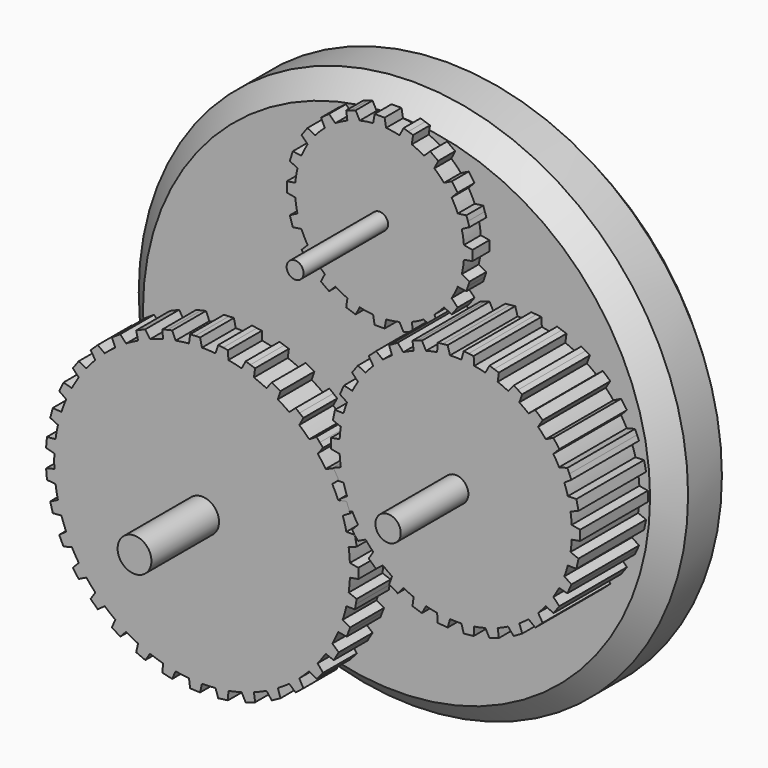
from build123d import *

# Parameters (mm, degrees)
F0_R      = 65
F1_DEPTH  = 20
F2_R      = 2
F3_DEPTH  = 5
F4_R      = 2
F5_DEPTH  = 30
F6_R      = 3
F7_DEPTH  = 20
F8_R      = 3
F9_DEPTH  = 40
F11_R     = 4
F12_DEPTH = 10
F13_R     = 4
F14_DEPTH = 40
F15_SIZE  = 5
F16_R     = 4
F17_DEPTH = 20
F18_DEPTH = 30
F19_W     = 40
F19_H     = 15
F20_DEPTH = 5
F21_W     = 8
F21_H     = 5
F22_DEPTH = 50
F24_DEPTH = 5
F26_DEPTH = 5
F27_W     = 10
F27_H     = 10
F28_DEPTH = 4
F29_DEPTH = 10
F30_R     = 2
F31_DEPTH = 4
F32_R     = 3
F33_DEPTH = 4


with BuildPart() as f1:
    # F0 (on Front) → F1 (new body)
    with BuildSketch(Plane.XZ):
        Circle(F0_R)
    extrude(amount=F1_DEPTH)

    # F15
    f15_edges = [f1.edges().sort_by_distance(p)[0] for p in [
        (-65, 0, 0),
        (65, -10, 0),
        (-65, -20, 0),
    ]]
    chamfer(f15_edges, length=F15_SIZE)

    # F16 (on face) → F17 (cut)
    with BuildSketch(Plane.XZ.offset(20)):
        with Locations((-30, -25)):
            Circle(F16_R)
    extrude(amount=-F17_DEPTH, mode=Mode.SUBTRACT)

    # F27 (on face) → F28 (cut)
    with BuildSketch(Plane(origin=(0, 0, 0), x_dir=(-1, 0, 0), z_dir=(0, 1, 0))):
        with Locations((-45, 0)):
            Rectangle(F27_W, F27_H)
        Polygon((-15.6698729811, -37.1410161514), (-24.3301270189, -32.1410161514), (-29.3301270189, -40.8012701892), (-20.6698729811, -45.8012701892), align=None)
        Polygon((24.3301270189, -32.1410161514), (15.6698729811, -37.1410161514), (20.6698729811, -45.8012701892), (29.3301270189, -40.8012701892), align=None)
        with Locations((45, 0)):
            Rectangle(F27_W, F27_H)
        Polygon((15.6698729811, 37.1410161514), (24.3301270189, 32.1410161514), (29.3301270189, 40.8012701892), (20.6698729811, 45.8012701892), align=None)
        Polygon((-24.3301270189, 32.1410161514), (-15.6698729811, 37.1410161514), (-20.6698729811, 45.8012701892), (-29.3301270189, 40.8012701892), align=None)
    extrude(amount=-F28_DEPTH, mode=Mode.SUBTRACT)


with BuildPart() as f3:
    # F2 (on face) → F3 (new body)
    with BuildSketch(Plane.XZ.offset(20)):
        with BuildLine():
            ThreePointArc((19.9409690564, 38.4645023307), (19.9852368153, 39.2316840258), (20, 40))
            ThreePointArc((20, 40), (19.9852368153, 40.7683159742), (19.9409690564, 41.5354976693))
            ThreePointArc((19.9409690564, 41.5354976693), (19.7537668119, 43.1286893008), (19.4394834369, 44.7017532586))
            ThreePointArc((19.4394834369, 44.7017532586), (19.0211303259, 46.1803398875), (18.4904936877, 47.6224433869))
            ThreePointArc((18.4904936877, 47.6224433869), (17.8201304838, 49.0798099948), (17.0351257359, 50.4787638185))
            ThreePointArc((17.0351257359, 50.4787638185), (16.1803398875, 51.7557050458), (15.230039966, 52.963251237))
            ThreePointArc((15.230039966, 52.963251237), (14.1421356237, 54.1421356237), (12.963251237, 55.230039966))
            ThreePointArc((12.963251237, 55.230039966), (11.7557050458, 56.1803398875), (10.4787638185, 57.0351257359))
            ThreePointArc((10.4787638185, 57.0351257359), (9.0798099948, 57.8201304838), (7.6224433869, 58.4904936877))
            ThreePointArc((7.6224433869, 58.4904936877), (6.1803398875, 59.0211303259), (4.7017532586, 59.4394834369))
            ThreePointArc((4.7017532586, 59.4394834369), (3.1286893008, 59.7537668119), (1.5354976693, 59.9409690564))
            ThreePointArc((1.5354976693, 59.9409690564), (0, 60), (-1.5354976693, 59.9409690564))
            ThreePointArc((-1.5354976693, 59.9409690564), (-3.1286893008, 59.7537668119), (-4.7017532586, 59.4394834369))
            ThreePointArc((-4.7017532586, 59.4394834369), (-6.1803398875, 59.0211303259), (-7.6224433869, 58.4904936877))
            ThreePointArc((-7.6224433869, 58.4904936877), (-9.0798099948, 57.8201304838), (-10.4787638185, 57.0351257359))
            ThreePointArc((-10.4787638185, 57.0351257359), (-11.7557050458, 56.1803398875), (-12.963251237, 55.230039966))
            ThreePointArc((-12.963251237, 55.230039966), (-14.1421356237, 54.1421356237), (-15.230039966, 52.963251237))
            ThreePointArc((-15.230039966, 52.963251237), (-16.1803398875, 51.7557050458), (-17.0351257359, 50.4787638185))
            ThreePointArc((-17.0351257359, 50.4787638185), (-17.8201304838, 49.0798099948), (-18.4904936877, 47.6224433869))
            ThreePointArc((-18.4904936877, 47.6224433869), (-19.0211303259, 46.1803398875), (-19.4394834369, 44.7017532586))
            ThreePointArc((-19.4394834369, 44.7017532586), (-19.7537668119, 43.1286893008), (-19.9409690564, 41.5354976693))
            ThreePointArc((-19.9409690564, 41.5354976693), (-20, 40), (-19.9409690564, 38.4645023307))
            ThreePointArc((-19.9409690564, 38.4645023307), (-19.7537668119, 36.8713106992), (-19.4394834369, 35.2982467414))
            ThreePointArc((-19.4394834369, 35.2982467414), (-19.0211303259, 33.8196601125), (-18.4904936877, 32.3775566131))
            ThreePointArc((-18.4904936877, 32.3775566131), (-17.8201304838, 30.9201900052), (-17.0351257359, 29.5212361815))
            ThreePointArc((-17.0351257359, 29.5212361815), (-16.1803398875, 28.2442949542), (-15.230039966, 27.036748763))
            ThreePointArc((-15.230039966, 27.036748763), (-14.1421356237, 25.8578643763), (-12.963251237, 24.769960034))
            ThreePointArc((-12.963251237, 24.769960034), (-11.7557050458, 23.8196601125), (-10.4787638185, 22.9648742641))
            ThreePointArc((-10.4787638185, 22.9648742641), (-9.0798099948, 22.1798695162), (-7.6224433869, 21.5095063123))
            ThreePointArc((-7.6224433869, 21.5095063123), (-6.1803398875, 20.9788696741), (-4.7017532586, 20.5605165631))
            ThreePointArc((-4.7017532586, 20.5605165631), (-3.1286893008, 20.2462331881), (-1.5354976693, 20.0590309436))
            ThreePointArc((-1.5354976693, 20.0590309436), (0, 20), (1.5354976693, 20.0590309436))
            ThreePointArc((1.5354976693, 20.0590309436), (3.1286893008, 20.2462331881), (4.7017532586, 20.5605165631))
            ThreePointArc((4.7017532586, 20.5605165631), (6.1803398875, 20.9788696741), (7.6224433869, 21.5095063123))
            ThreePointArc((7.6224433869, 21.5095063123), (9.0798099948, 22.1798695162), (10.4787638185, 22.9648742641))
            ThreePointArc((10.4787638185, 22.9648742641), (11.7557050458, 23.8196601125), (12.963251237, 24.769960034))
            ThreePointArc((12.963251237, 24.769960034), (14.1421356237, 25.8578643763), (15.230039966, 27.036748763))
            ThreePointArc((15.230039966, 27.036748763), (16.1803398875, 28.2442949542), (17.0351257359, 29.5212361815))
            ThreePointArc((17.0351257359, 29.5212361815), (17.8201304838, 30.9201900052), (18.4904936877, 32.3775566131))
            ThreePointArc((18.4904936877, 32.3775566131), (19.0211303259, 33.8196601125), (19.4394834369, 35.2982467414))
            ThreePointArc((19.4394834369, 35.2982467414), (19.7537668119, 36.8713106992), (19.9409690564, 38.4645023307))
        make_face()
        with Locations((0, 40)):
            Circle(F2_R, mode=Mode.SUBTRACT)
        with BuildLine():
            ThreePointArc((19.9409690564, 41.5354976693), (19.9852368153, 40.7683159742), (20, 40))
            ThreePointArc((20, 40), (19.9852368153, 39.2316840258), (19.9409690564, 38.4645023307))
            Line((19.9409690564, 38.4645023307), (21.9684390888, 38.822))
            Line((21.9684390888, 38.822), (21.9684390888, 40))
            Line((21.9684390888, 40), (21.9684390888, 41.178))
            Line((21.9684390888, 41.178), (19.9409690564, 41.5354976693))
        make_face()
        with BuildLine():
            ThreePointArc((18.4904936877, 47.6224433869), (19.0211303259, 46.1803398875), (19.4394834369, 44.7017532586))
            Line((19.4394834369, 44.7017532586), (21.2572491676, 45.6682764421))
            Line((21.2572491676, 45.6682764421), (20.8932271483, 46.7886210183))
            Line((20.8932271483, 46.7886210183), (20.5292051289, 47.9089655945))
            Line((20.5292051289, 47.9089655945), (18.4904936877, 47.6224433869))
        make_face()
        with BuildLine():
            Line((21.2572491676, 34.3317235579), (19.4394834369, 35.2982467414))
            ThreePointArc((19.4394834369, 35.2982467414), (19.0211303259, 33.8196601125), (18.4904936877, 32.3775566131))
            Line((18.4904936877, 32.3775566131), (20.5292051289, 32.0910344055))
            Line((20.5292051289, 32.0910344055), (20.8932271483, 33.2113789817))
            Line((20.8932271483, 33.2113789817), (21.2572491676, 34.3317235579))
        make_face()
        with BuildLine():
            ThreePointArc((15.230039966, 52.963251237), (16.1803398875, 51.7557050458), (17.0351257359, 50.4787638185))
            Line((17.0351257359, 50.4787638185), (18.46525159, 51.9597024929))
            Line((18.46525159, 51.9597024929), (17.7728405628, 52.9127245123))
            Line((17.7728405628, 52.9127245123), (17.0804295356, 53.8657465317))
            Line((17.0804295356, 53.8657465317), (15.230039966, 52.963251237))
        make_face()
        with BuildLine():
            Line((18.46525159, 28.0402975071), (17.0351257359, 29.5212361815))
            ThreePointArc((17.0351257359, 29.5212361815), (16.1803398875, 28.2442949542), (15.230039966, 27.036748763))
            Line((15.230039966, 27.036748763), (17.0804295356, 26.1342534683))
            Line((17.0804295356, 26.1342534683), (17.7728405628, 27.0872754877))
            Line((17.7728405628, 27.0872754877), (18.46525159, 28.0402975071))
        make_face()
        with BuildLine():
            ThreePointArc((10.4787638185, 57.0351257359), (11.7557050458, 56.1803398875), (12.963251237, 55.230039966))
            Line((12.963251237, 55.230039966), (13.8657465317, 57.0804295356))
            Line((13.8657465317, 57.0804295356), (12.9127245123, 57.7728405628))
            Line((12.9127245123, 57.7728405628), (11.9597024929, 58.46525159))
            Line((11.9597024929, 58.46525159), (10.4787638185, 57.0351257359))
        make_face()
        with BuildLine():
            Line((13.8657465317, 22.9195704644), (12.963251237, 24.769960034))
            ThreePointArc((12.963251237, 24.769960034), (11.7557050458, 23.8196601125), (10.4787638185, 22.9648742641))
            Line((10.4787638185, 22.9648742641), (11.9597024929, 21.53474841))
            Line((11.9597024929, 21.53474841), (12.9127245123, 22.2271594372))
            Line((12.9127245123, 22.2271594372), (13.8657465317, 22.9195704644))
        make_face()
        with BuildLine():
            ThreePointArc((4.7017532586, 59.4394834369), (6.1803398875, 59.0211303259), (7.6224433869, 58.4904936877))
            Line((7.6224433869, 58.4904936877), (7.9089655945, 60.5292051289))
            Line((7.9089655945, 60.5292051289), (6.7886210183, 60.8932271483))
            Line((6.7886210183, 60.8932271483), (5.6682764421, 61.2572491676))
            Line((5.6682764421, 61.2572491676), (4.7017532586, 59.4394834369))
        make_face()
        with BuildLine():
            Line((7.9089655945, 19.4707948711), (7.6224433869, 21.5095063123))
            ThreePointArc((7.6224433869, 21.5095063123), (6.1803398875, 20.9788696741), (4.7017532586, 20.5605165631))
            Line((4.7017532586, 20.5605165631), (5.6682764421, 18.7427508324))
            Line((5.6682764421, 18.7427508324), (6.7886210183, 19.1067728517))
            Line((6.7886210183, 19.1067728517), (7.9089655945, 19.4707948711))
        make_face()
        with BuildLine():
            ThreePointArc((-1.5354976693, 59.9409690564), (0, 60), (1.5354976693, 59.9409690564))
            Line((1.5354976693, 59.9409690564), (1.178, 61.9684390888))
            Line((1.178, 61.9684390888), (0, 61.9684390888))
            Line((0, 61.9684390888), (-1.178, 61.9684390888))
            Line((-1.178, 61.9684390888), (-1.5354976693, 59.9409690564))
        make_face()
        with BuildLine():
            Line((1.178, 18.0315609112), (1.5354976693, 20.0590309436))
            ThreePointArc((1.5354976693, 20.0590309436), (0, 20), (-1.5354976693, 20.0590309436))
            Line((-1.5354976693, 20.0590309436), (-1.178, 18.0315609112))
            Line((-1.178, 18.0315609112), (0, 18.0315609112))
            Line((0, 18.0315609112), (1.178, 18.0315609112))
        make_face()
        with BuildLine():
            ThreePointArc((-7.6224433869, 58.4904936877), (-6.1803398875, 59.0211303259), (-4.7017532586, 59.4394834369))
            Line((-4.7017532586, 59.4394834369), (-5.6682764421, 61.2572491676))
            Line((-5.6682764421, 61.2572491676), (-6.7886210183, 60.8932271483))
            Line((-6.7886210183, 60.8932271483), (-7.9089655945, 60.5292051289))
            Line((-7.9089655945, 60.5292051289), (-7.6224433869, 58.4904936877))
        make_face()
        with BuildLine():
            Line((-5.6682764421, 18.7427508324), (-4.7017532586, 20.5605165631))
            ThreePointArc((-4.7017532586, 20.5605165631), (-6.1803398875, 20.9788696741), (-7.6224433869, 21.5095063123))
            Line((-7.6224433869, 21.5095063123), (-7.9089655945, 19.4707948711))
            Line((-7.9089655945, 19.4707948711), (-6.7886210183, 19.1067728517))
            Line((-6.7886210183, 19.1067728517), (-5.6682764421, 18.7427508324))
        make_face()
        with BuildLine():
            ThreePointArc((-12.963251237, 55.230039966), (-11.7557050458, 56.1803398875), (-10.4787638185, 57.0351257359))
            Line((-10.4787638185, 57.0351257359), (-11.9597024929, 58.46525159))
            Line((-11.9597024929, 58.46525159), (-12.9127245123, 57.7728405628))
            Line((-12.9127245123, 57.7728405628), (-13.8657465317, 57.0804295356))
            Line((-13.8657465317, 57.0804295356), (-12.963251237, 55.230039966))
        make_face()
        with BuildLine():
            Line((-11.9597024929, 21.53474841), (-10.4787638185, 22.9648742641))
            ThreePointArc((-10.4787638185, 22.9648742641), (-11.7557050458, 23.8196601125), (-12.963251237, 24.769960034))
            Line((-12.963251237, 24.769960034), (-13.8657465317, 22.9195704644))
            Line((-13.8657465317, 22.9195704644), (-12.9127245123, 22.2271594372))
            Line((-12.9127245123, 22.2271594372), (-11.9597024929, 21.53474841))
        make_face()
        with BuildLine():
            ThreePointArc((-17.0351257359, 50.4787638185), (-16.1803398875, 51.7557050458), (-15.230039966, 52.963251237))
            Line((-15.230039966, 52.963251237), (-17.0804295356, 53.8657465317))
            Line((-17.0804295356, 53.8657465317), (-17.7728405628, 52.9127245123))
            Line((-17.7728405628, 52.9127245123), (-18.46525159, 51.9597024929))
            Line((-18.46525159, 51.9597024929), (-17.0351257359, 50.4787638185))
        make_face()
        with BuildLine():
            Line((-17.0804295356, 26.1342534683), (-15.230039966, 27.036748763))
            ThreePointArc((-15.230039966, 27.036748763), (-16.1803398875, 28.2442949542), (-17.0351257359, 29.5212361815))
            Line((-17.0351257359, 29.5212361815), (-18.46525159, 28.0402975071))
            Line((-18.46525159, 28.0402975071), (-17.7728405628, 27.0872754877))
            Line((-17.7728405628, 27.0872754877), (-17.0804295356, 26.1342534683))
        make_face()
        with BuildLine():
            ThreePointArc((-19.4394834369, 44.7017532586), (-19.0211303259, 46.1803398875), (-18.4904936877, 47.6224433869))
            Line((-18.4904936877, 47.6224433869), (-20.5292051289, 47.9089655945))
            Line((-20.5292051289, 47.9089655945), (-20.8932271483, 46.7886210183))
            Line((-20.8932271483, 46.7886210183), (-21.2572491676, 45.6682764421))
            Line((-21.2572491676, 45.6682764421), (-19.4394834369, 44.7017532586))
        make_face()
        with BuildLine():
            Line((-20.5292051289, 32.0910344055), (-18.4904936877, 32.3775566131))
            ThreePointArc((-18.4904936877, 32.3775566131), (-19.0211303259, 33.8196601125), (-19.4394834369, 35.2982467414))
            Line((-19.4394834369, 35.2982467414), (-21.2572491676, 34.3317235579))
            Line((-21.2572491676, 34.3317235579), (-20.8932271483, 33.2113789817))
            Line((-20.8932271483, 33.2113789817), (-20.5292051289, 32.0910344055))
        make_face()
        with BuildLine():
            ThreePointArc((-19.9409690564, 38.4645023307), (-20, 40), (-19.9409690564, 41.5354976693))
            Line((-19.9409690564, 41.5354976693), (-21.9684390888, 41.178))
            Line((-21.9684390888, 41.178), (-21.9684390888, 40))
            Line((-21.9684390888, 40), (-21.9684390888, 38.822))
            Line((-21.9684390888, 38.822), (-19.9409690564, 38.4645023307))
        make_face()
    extrude(amount=F3_DEPTH)


with BuildPart() as f5:
    # F4 (on face) → F5 (new body)
    with BuildSketch(Plane.XZ.offset(20)):
        with Locations((0, 40)):
            Circle(F4_R)
    extrude(amount=F5_DEPTH)


with BuildPart() as f7:
    # F6 (on face) → F7 (new body)
    with BuildSketch(Plane.XZ.offset(20)):
        with BuildLine():
            ThreePointArc((57.4573687459, -1.5306539614), (57.4893401204, -0.765623761), (57.5, 0))
            ThreePointArc((57.5, 0), (57.4893401204, 0.765623761), (57.4573687459, 1.5306539614))
            ThreePointArc((57.4573687459, 1.5306539614), (57.3493521226, 2.8745327399), (57.1756002145, 4.2115024615))
            ThreePointArc((57.1756002145, 4.2115024615), (56.8990590202, 5.7175714975), (56.5391185081, 7.2059134613))
            ThreePointArc((56.5391185081, 7.2059134613), (56.1540541981, 8.4979673453), (55.7061275506, 9.7695960177))
            ThreePointArc((55.7061275506, 9.7695960177), (55.1225000852, 11.1852576846), (54.4609814427, 12.5662399651))
            ThreePointArc((54.4609814427, 12.5662399651), (53.8156986041, 13.75), (53.1131737612, 14.9007113483))
            ThreePointArc((53.1131737612, 14.9007113483), (52.2479673453, 16.164094438), (51.3137821114, 17.3773614829))
            ThreePointArc((51.3137821114, 17.3773614829), (50.4364827006, 18.4010916749), (49.510063369, 19.3805940914))
            ThreePointArc((49.510063369, 19.3805940914), (48.4010916749, 20.4364827006), (47.235068227, 21.4290089181))
            ThreePointArc((47.235068227, 21.4290089181), (46.164094438, 22.2479673453), (45.054269588, 23.0134518744))
            ThreePointArc((45.054269588, 23.0134518744), (43.75, 23.8156986041), (42.403099158, 24.5441058358))
            ThreePointArc((42.403099158, 24.5441058358), (41.1852576846, 25.1225000852), (39.9405319875, 25.6405113796))
            ThreePointArc((39.9405319875, 25.6405113796), (38.4979673453, 26.1540541981), (37.0290551391, 26.5865075527))
            ThreePointArc((37.0290551391, 26.5865075527), (35.7175714975, 26.8990590202), (34.3923454392, 27.1469575007))
            ThreePointArc((34.3923454392, 27.1469575007), (32.8745327399, 27.3493521226), (31.3478076815, 27.4669513134))
            ThreePointArc((31.3478076815, 27.4669513134), (30, 27.5), (28.6521923185, 27.4669513134))
            ThreePointArc((28.6521923185, 27.4669513134), (27.1254672601, 27.3493521226), (25.6076545608, 27.1469575007))
            ThreePointArc((25.6076545608, 27.1469575007), (24.2824285025, 26.8990590202), (22.9709448609, 26.5865075527))
            ThreePointArc((22.9709448609, 26.5865075527), (21.5020326547, 26.1540541981), (20.0594680125, 25.6405113796))
            ThreePointArc((20.0594680125, 25.6405113796), (18.8147423154, 25.1225000852), (17.596900842, 24.5441058358))
            ThreePointArc((17.596900842, 24.5441058358), (16.25, 23.8156986041), (14.945730412, 23.0134518744))
            ThreePointArc((14.945730412, 23.0134518744), (13.835905562, 22.2479673453), (12.764931773, 21.4290089181))
            ThreePointArc((12.764931773, 21.4290089181), (11.5989083251, 20.4364827006), (10.489936631, 19.3805940914))
            ThreePointArc((10.489936631, 19.3805940914), (9.5635172994, 18.4010916749), (8.6862178886, 17.3773614829))
            ThreePointArc((8.6862178886, 17.3773614829), (7.7520326547, 16.164094438), (6.8868262388, 14.9007113483))
            ThreePointArc((6.8868262388, 14.9007113483), (6.1843013959, 13.75), (5.5390185573, 12.5662399651))
            ThreePointArc((5.5390185573, 12.5662399651), (4.8774999148, 11.1852576846), (4.2938724494, 9.7695960177))
            ThreePointArc((4.2938724494, 9.7695960177), (3.8459458019, 8.4979673453), (3.4608814919, 7.2059134613))
            ThreePointArc((3.4608814919, 7.2059134613), (3.1009409798, 5.7175714975), (2.8243997855, 4.2115024615))
            ThreePointArc((2.8243997855, 4.2115024615), (2.6506478774, 2.8745327399), (2.5426312541, 1.5306539614))
            ThreePointArc((2.5426312541, 1.5306539614), (2.5, 0), (2.5426312541, -1.5306539614))
            ThreePointArc((2.5426312541, -1.5306539614), (2.6506478774, -2.8745327399), (2.8243997855, -4.2115024615))
            ThreePointArc((2.8243997855, -4.2115024615), (3.1009409798, -5.7175714975), (3.4608814919, -7.2059134613))
            ThreePointArc((3.4608814919, -7.2059134613), (3.8459458019, -8.4979673453), (4.2938724494, -9.7695960177))
            ThreePointArc((4.2938724494, -9.7695960177), (4.8774999148, -11.1852576846), (5.5390185573, -12.5662399651))
            ThreePointArc((5.5390185573, -12.5662399651), (6.1843013959, -13.75), (6.8868262388, -14.9007113483))
            ThreePointArc((6.8868262388, -14.9007113483), (7.7520326547, -16.164094438), (8.6862178886, -17.3773614829))
            ThreePointArc((8.6862178886, -17.3773614829), (9.5635172994, -18.4010916749), (10.489936631, -19.3805940914))
            ThreePointArc((10.489936631, -19.3805940914), (11.5989083251, -20.4364827006), (12.764931773, -21.4290089181))
            ThreePointArc((12.764931773, -21.4290089181), (13.835905562, -22.2479673453), (14.945730412, -23.0134518744))
            ThreePointArc((14.945730412, -23.0134518744), (16.25, -23.8156986041), (17.596900842, -24.5441058358))
            ThreePointArc((17.596900842, -24.5441058358), (18.8147423154, -25.1225000852), (20.0594680125, -25.6405113796))
            ThreePointArc((20.0594680125, -25.6405113796), (21.5020326547, -26.1540541981), (22.9709448609, -26.5865075527))
            ThreePointArc((22.9709448609, -26.5865075527), (24.2824285025, -26.8990590202), (25.6076545608, -27.1469575007))
            ThreePointArc((25.6076545608, -27.1469575007), (27.1254672601, -27.3493521226), (28.6521923185, -27.4669513134))
            ThreePointArc((28.6521923185, -27.4669513134), (30, -27.5), (31.3478076815, -27.4669513134))
            ThreePointArc((31.3478076815, -27.4669513134), (32.8745327399, -27.3493521226), (34.3923454392, -27.1469575007))
            ThreePointArc((34.3923454392, -27.1469575007), (35.7175714975, -26.8990590202), (37.0290551391, -26.5865075527))
            ThreePointArc((37.0290551391, -26.5865075527), (38.4979673453, -26.1540541981), (39.9405319875, -25.6405113796))
            ThreePointArc((39.9405319875, -25.6405113796), (41.1852576846, -25.1225000852), (42.403099158, -24.5441058358))
            ThreePointArc((42.403099158, -24.5441058358), (43.75, -23.8156986041), (45.054269588, -23.0134518744))
            ThreePointArc((45.054269588, -23.0134518744), (46.164094438, -22.2479673453), (47.235068227, -21.4290089181))
            ThreePointArc((47.235068227, -21.4290089181), (48.4010916749, -20.4364827006), (49.510063369, -19.3805940914))
            ThreePointArc((49.510063369, -19.3805940914), (50.4364827006, -18.4010916749), (51.3137821114, -17.3773614829))
            ThreePointArc((51.3137821114, -17.3773614829), (52.2479673453, -16.164094438), (53.1131737612, -14.9007113483))
            ThreePointArc((53.1131737612, -14.9007113483), (53.8156986041, -13.75), (54.4609814427, -12.5662399651))
            ThreePointArc((54.4609814427, -12.5662399651), (55.1225000852, -11.1852576846), (55.7061275506, -9.7695960177))
            ThreePointArc((55.7061275506, -9.7695960177), (56.1540541981, -8.4979673453), (56.5391185081, -7.2059134613))
            ThreePointArc((56.5391185081, -7.2059134613), (56.8990590202, -5.7175714975), (57.1756002145, -4.2115024615))
            ThreePointArc((57.1756002145, -4.2115024615), (57.3493521226, -2.8745327399), (57.4573687459, -1.5306539614))
        make_face()
        with Locations((30, 0)):
            Circle(F6_R, mode=Mode.SUBTRACT)
        with BuildLine():
            ThreePointArc((57.4573687459, 1.5306539614), (57.4893401204, 0.765623761), (57.5, 0))
            ThreePointArc((57.5, 0), (57.4893401204, -0.765623761), (57.4573687459, -1.5306539614))
            Line((57.4573687459, -1.5306539614), (59.4573687459, -1.178))
            Line((59.4573687459, -1.178), (59.4573687459, 0))
            Line((59.4573687459, 0), (59.4573687459, 1.178))
            Line((59.4573687459, 1.178), (57.4573687459, 1.5306539614))
        make_face()
        with BuildLine():
            ThreePointArc((56.5391185081, 7.2059134613), (56.8990590202, 5.7175714975), (57.1756002145, 4.2115024615))
            Line((57.1756002145, 4.2115024615), (59.0585745346, 4.9722734693))
            Line((59.0585745346, 4.9722734693), (58.8136545628, 6.124531343))
            Line((58.8136545628, 6.124531343), (58.568734591, 7.2767892167))
            Line((58.568734591, 7.2767892167), (56.5391185081, 7.2059134613))
        make_face()
        with BuildLine():
            Line((59.0585745346, -4.9722734693), (57.1756002145, -4.2115024615))
            ThreePointArc((57.1756002145, -4.2115024615), (56.8990590202, -5.7175714975), (56.5391185081, -7.2059134613))
            Line((56.5391185081, -7.2059134613), (58.568734591, -7.2767892167))
            Line((58.568734591, -7.2767892167), (58.8136545628, -6.124531343))
            Line((58.8136545628, -6.124531343), (59.0585745346, -4.9722734693))
        make_face()
        with BuildLine():
            ThreePointArc((54.4609814427, 12.5662399651), (55.1225000852, 11.1852576846), (55.7061275506, 9.7695960177))
            Line((55.7061275506, 9.7695960177), (57.3897811775, 10.9052347285))
            Line((57.3897811775, 10.9052347285), (56.910645412, 11.9813912776))
            Line((56.910645412, 11.9813912776), (56.4315096464, 13.0575478267))
            Line((56.4315096464, 13.0575478267), (54.4609814427, 12.5662399651))
        make_face()
        with BuildLine():
            Line((57.3897811775, -10.9052347285), (55.7061275506, -9.7695960177))
            ThreePointArc((55.7061275506, -9.7695960177), (55.1225000852, -11.1852576846), (54.4609814427, -12.5662399651))
            Line((54.4609814427, -12.5662399651), (56.4315096464, -13.0575478267))
            Line((56.4315096464, -13.0575478267), (56.910645412, -11.9813912776))
            Line((56.910645412, -11.9813912776), (57.3897811775, -10.9052347285))
        make_face()
        with BuildLine():
            ThreePointArc((51.3137821114, 17.3773614829), (52.2479673453, 16.164094438), (53.1131737612, 14.9007113483))
            Line((53.1131737612, 14.9007113483), (54.5239229522, 16.3615849008))
            Line((54.5239229522, 16.3615849008), (53.831511925, 17.3146069202))
            Line((53.831511925, 17.3146069202), (53.1391008978, 18.2676289396))
            Line((53.1391008978, 18.2676289396), (51.3137821114, 17.3773614829))
        make_face()
        with BuildLine():
            Line((54.5239229522, -16.3615849008), (53.1131737612, -14.9007113483))
            ThreePointArc((53.1131737612, -14.9007113483), (52.2479673453, -16.164094438), (51.3137821114, -17.3773614829))
            Line((51.3137821114, -17.3773614829), (53.1391008978, -18.2676289396))
            Line((53.1391008978, -18.2676289396), (53.831511925, -17.3146069202))
            Line((53.831511925, -17.3146069202), (54.5239229522, -16.3615849008))
        make_face()
        with BuildLine():
            ThreePointArc((47.235068227, 21.4290089181), (48.4010916749, 20.4364827006), (49.510063369, 19.3805940914))
            Line((49.510063369, 19.3805940914), (50.5862516151, 21.1028553014))
            Line((50.5862516151, 21.1028553014), (49.7108270107, 21.8910911557))
            Line((49.7108270107, 21.8910911557), (48.8354024063, 22.67932701))
            Line((48.8354024063, 22.67932701), (47.235068227, 21.4290089181))
        make_face()
        with BuildLine():
            Line((50.5862516151, -21.1028553014), (49.510063369, -19.3805940914))
            ThreePointArc((49.510063369, -19.3805940914), (48.4010916749, -20.4364827006), (47.235068227, -21.4290089181))
            Line((47.235068227, -21.4290089181), (48.8354024063, -22.67932701))
            Line((48.8354024063, -22.67932701), (49.7108270107, -21.8910911557))
            Line((49.7108270107, -21.8910911557), (50.5862516151, -21.1028553014))
        make_face()
        with BuildLine():
            ThreePointArc((42.403099158, 24.5441058358), (43.75, 23.8156986041), (45.054269588, 23.0134518744))
            Line((45.054269588, 23.0134518744), (45.7488622986, 24.9218296626))
            Line((45.7488622986, 24.9218296626), (44.728684373, 25.5108296626))
            Line((44.728684373, 25.5108296626), (43.7085064473, 26.0998296626))
            Line((43.7085064473, 26.0998296626), (42.403099158, 24.5441058358))
        make_face()
        with BuildLine():
            Line((45.7488622986, -24.9218296626), (45.054269588, -23.0134518744))
            ThreePointArc((45.054269588, -23.0134518744), (43.75, -23.8156986041), (42.403099158, -24.5441058358))
            Line((42.403099158, -24.5441058358), (43.7085064473, -26.0998296626))
            Line((43.7085064473, -26.0998296626), (44.728684373, -25.5108296626))
            Line((44.728684373, -25.5108296626), (45.7488622986, -24.9218296626))
        make_face()
        with BuildLine():
            ThreePointArc((37.0290551391, 26.5865075527), (38.4979673453, 26.1540541981), (39.9405319875, 25.6405113796))
            Line((39.9405319875, 25.6405113796), (40.2231721283, 27.6516004794))
            Line((40.2231721283, 27.6516004794), (39.1028275521, 28.0156224987))
            Line((39.1028275521, 28.0156224987), (37.9824829759, 28.3796445181))
            Line((37.9824829759, 28.3796445181), (37.0290551391, 26.5865075527))
        make_face()
        with BuildLine():
            Line((40.2231721283, -27.6516004794), (39.9405319875, -25.6405113796))
            ThreePointArc((39.9405319875, -25.6405113796), (38.4979673453, -26.1540541981), (37.0290551391, -26.5865075527))
            Line((37.0290551391, -26.5865075527), (37.9824829759, -28.3796445181))
            Line((37.9824829759, -28.3796445181), (39.1028275521, -28.0156224987))
            Line((39.1028275521, -28.0156224987), (40.2231721283, -27.6516004794))
        make_face()
        with BuildLine():
            ThreePointArc((31.3478076815, 27.4669513134), (32.8745327399, 27.3493521226), (34.3923454392, 27.1469575007))
            Line((34.3923454392, 27.1469575007), (34.2506802797, 29.172863668))
            Line((34.2506802797, 29.172863668), (33.0791334869, 29.2959981978))
            Line((33.0791334869, 29.2959981978), (31.9075866942, 29.4191327275))
            Line((31.9075866942, 29.4191327275), (31.3478076815, 27.4669513134))
        make_face()
        with BuildLine():
            Line((34.2506802797, -29.172863668), (34.3923454392, -27.1469575007))
            ThreePointArc((34.3923454392, -27.1469575007), (32.8745327399, -27.3493521226), (31.3478076815, -27.4669513134))
            Line((31.3478076815, -27.4669513134), (31.9075866942, -29.4191327275))
            Line((31.9075866942, -29.4191327275), (33.0791334869, -29.2959981978))
            Line((33.0791334869, -29.2959981978), (34.2506802797, -29.172863668))
        make_face()
        with BuildLine():
            ThreePointArc((25.6076545608, 27.1469575007), (27.1254672601, 27.3493521226), (28.6521923185, 27.4669513134))
            Line((28.6521923185, 27.4669513134), (28.0924133058, 29.4191327275))
            Line((28.0924133058, 29.4191327275), (26.9208665131, 29.2959981978))
            Line((26.9208665131, 29.2959981978), (25.7493197203, 29.172863668))
            Line((25.7493197203, 29.172863668), (25.6076545608, 27.1469575007))
        make_face()
        with BuildLine():
            Line((28.0924133058, -29.4191327275), (28.6521923185, -27.4669513134))
            ThreePointArc((28.6521923185, -27.4669513134), (27.1254672601, -27.3493521226), (25.6076545608, -27.1469575007))
            Line((25.6076545608, -27.1469575007), (25.7493197203, -29.172863668))
            Line((25.7493197203, -29.172863668), (26.9208665131, -29.2959981978))
            Line((26.9208665131, -29.2959981978), (28.0924133058, -29.4191327275))
        make_face()
        with BuildLine():
            ThreePointArc((20.0594680125, 25.6405113796), (21.5020326547, 26.1540541981), (22.9709448609, 26.5865075527))
            Line((22.9709448609, 26.5865075527), (22.0175170241, 28.3796445181))
            Line((22.0175170241, 28.3796445181), (20.8971724479, 28.0156224987))
            Line((20.8971724479, 28.0156224987), (19.7768278717, 27.6516004794))
            Line((19.7768278717, 27.6516004794), (20.0594680125, 25.6405113796))
        make_face()
        with BuildLine():
            Line((22.0175170241, -28.3796445181), (22.9709448609, -26.5865075527))
            ThreePointArc((22.9709448609, -26.5865075527), (21.5020326547, -26.1540541981), (20.0594680125, -25.6405113796))
            Line((20.0594680125, -25.6405113796), (19.7768278717, -27.6516004794))
            Line((19.7768278717, -27.6516004794), (20.8971724479, -28.0156224987))
            Line((20.8971724479, -28.0156224987), (22.0175170241, -28.3796445181))
        make_face()
        with BuildLine():
            ThreePointArc((14.945730412, 23.0134518744), (16.25, 23.8156986041), (17.596900842, 24.5441058358))
            Line((17.596900842, 24.5441058358), (16.2914935527, 26.0998296626))
            Line((16.2914935527, 26.0998296626), (15.271315627, 25.5108296626))
            Line((15.271315627, 25.5108296626), (14.2511377014, 24.9218296626))
            Line((14.2511377014, 24.9218296626), (14.945730412, 23.0134518744))
        make_face()
        with BuildLine():
            Line((16.2914935527, -26.0998296626), (17.596900842, -24.5441058358))
            ThreePointArc((17.596900842, -24.5441058358), (16.25, -23.8156986041), (14.945730412, -23.0134518744))
            Line((14.945730412, -23.0134518744), (14.2511377014, -24.9218296626))
            Line((14.2511377014, -24.9218296626), (15.271315627, -25.5108296626))
            Line((15.271315627, -25.5108296626), (16.2914935527, -26.0998296626))
        make_face()
        with BuildLine():
            ThreePointArc((10.489936631, 19.3805940914), (11.5989083251, 20.4364827006), (12.764931773, 21.4290089181))
            Line((12.764931773, 21.4290089181), (11.1645975937, 22.67932701))
            Line((11.1645975937, 22.67932701), (10.2891729893, 21.8910911557))
            Line((10.2891729893, 21.8910911557), (9.4137483849, 21.1028553014))
            Line((9.4137483849, 21.1028553014), (10.489936631, 19.3805940914))
        make_face()
        with BuildLine():
            Line((11.1645975937, -22.67932701), (12.764931773, -21.4290089181))
            ThreePointArc((12.764931773, -21.4290089181), (11.5989083251, -20.4364827006), (10.489936631, -19.3805940914))
            Line((10.489936631, -19.3805940914), (9.4137483849, -21.1028553014))
            Line((9.4137483849, -21.1028553014), (10.2891729893, -21.8910911557))
            Line((10.2891729893, -21.8910911557), (11.1645975937, -22.67932701))
        make_face()
        with BuildLine():
            ThreePointArc((6.8868262388, 14.9007113483), (7.7520326547, 16.164094438), (8.6862178886, 17.3773614829))
            Line((8.6862178886, 17.3773614829), (6.8608991022, 18.2676289396))
            Line((6.8608991022, 18.2676289396), (6.168488075, 17.3146069202))
            Line((6.168488075, 17.3146069202), (5.4760770478, 16.3615849008))
            Line((5.4760770478, 16.3615849008), (6.8868262388, 14.9007113483))
        make_face()
        with BuildLine():
            Line((6.8608991022, -18.2676289396), (8.6862178886, -17.3773614829))
            ThreePointArc((8.6862178886, -17.3773614829), (7.7520326547, -16.164094438), (6.8868262388, -14.9007113483))
            Line((6.8868262388, -14.9007113483), (5.4760770478, -16.3615849008))
            Line((5.4760770478, -16.3615849008), (6.168488075, -17.3146069202))
            Line((6.168488075, -17.3146069202), (6.8608991022, -18.2676289396))
        make_face()
        with BuildLine():
            ThreePointArc((4.2938724494, 9.7695960177), (4.8774999148, 11.1852576846), (5.5390185573, 12.5662399651))
            Line((5.5390185573, 12.5662399651), (3.5684903536, 13.0575478267))
            Line((3.5684903536, 13.0575478267), (3.089354588, 11.9813912776))
            Line((3.089354588, 11.9813912776), (2.6102188225, 10.9052347285))
            Line((2.6102188225, 10.9052347285), (4.2938724494, 9.7695960177))
        make_face()
        with BuildLine():
            Line((3.5684903536, -13.0575478267), (5.5390185573, -12.5662399651))
            ThreePointArc((5.5390185573, -12.5662399651), (4.8774999148, -11.1852576846), (4.2938724494, -9.7695960177))
            Line((4.2938724494, -9.7695960177), (2.6102188225, -10.9052347285))
            Line((2.6102188225, -10.9052347285), (3.089354588, -11.9813912776))
            Line((3.089354588, -11.9813912776), (3.5684903536, -13.0575478267))
        make_face()
        with BuildLine():
            ThreePointArc((2.8243997855, 4.2115024615), (3.1009409798, 5.7175714975), (3.4608814919, 7.2059134613))
            Line((3.4608814919, 7.2059134613), (1.431265409, 7.2767892167))
            Line((1.431265409, 7.2767892167), (1.1863454372, 6.124531343))
            Line((1.1863454372, 6.124531343), (0.9414254654, 4.9722734693))
            Line((0.9414254654, 4.9722734693), (2.8243997855, 4.2115024615))
        make_face()
        with BuildLine():
            Line((1.431265409, -7.2767892167), (3.4608814919, -7.2059134613))
            ThreePointArc((3.4608814919, -7.2059134613), (3.1009409798, -5.7175714975), (2.8243997855, -4.2115024615))
            Line((2.8243997855, -4.2115024615), (0.9414254654, -4.9722734693))
            Line((0.9414254654, -4.9722734693), (1.1863454372, -6.124531343))
            Line((1.1863454372, -6.124531343), (1.431265409, -7.2767892167))
        make_face()
        with BuildLine():
            ThreePointArc((2.5426312541, -1.5306539614), (2.5, 0), (2.5426312541, 1.5306539614))
            Line((2.5426312541, 1.5306539614), (0.5426312541, 1.178))
            Line((0.5426312541, 1.178), (0.5426312541, 0))
            Line((0.5426312541, 0), (0.5426312541, -1.178))
            Line((0.5426312541, -1.178), (2.5426312541, -1.5306539614))
        make_face()
    extrude(amount=F7_DEPTH)


with BuildPart() as f9:
    # F8 (on face) → F9 (new body)
    with BuildSketch(Plane.XZ.offset(20)):
        with Locations((30, 0)):
            Circle(F8_R)
    extrude(amount=F9_DEPTH)


with BuildPart() as f12:
    # F11 (on offset) → F12 (new body)
    with BuildSketch(Plane.XZ.offset(30)):
        with BuildLine():
            ThreePointArc((4.9665139591, -26.5306539614), (4.9916274884, -25.7655101019), (5, -25))
            ThreePointArc((5, -25), (4.9916274884, -24.2344898981), (4.9665139591, -23.4693460386))
            ThreePointArc((4.9665139591, -23.4693460386), (4.8591002898, -21.8626241884), (4.6778965128, -20.2625435681))
            ThreePointArc((4.6778965128, -20.2625435681), (4.437535601, -18.750508682), (4.1312788761, -17.250432123))
            ThreePointArc((4.1312788761, -17.250432123), (3.7387001244, -15.6887104052), (3.2747029396, -14.1466989225))
            ThreePointArc((3.2747029396, -14.1466989225), (2.7682204724, -12.7018811572), (2.1990364068, -11.2805956953))
            ThreePointArc((2.1990364068, -11.2805956953), (1.5339103766, -9.8140691309), (0.8020330354, -8.3796883036))
            ThreePointArc((0.8020330354, -8.3796883036), (0.0457077761, -7.0485252908), (-0.7681095861, -5.7517122104))
            ThreePointArc((-0.7681095861, -5.7517122104), (-1.6844051969, -4.4275161698), (-2.6606395546, -3.1468681779))
            ThreePointArc((-2.6606395546, -3.1468681779), (-3.6424986899, -1.9721445921), (-4.674792589, -0.8414845325))
            ThreePointArc((-4.674792589, -0.8414845325), (-5.8128072855, 0.297820234), (-7.0020216842, 1.3835743102))
            ThreePointArc((-7.0020216842, 1.3835743102), (-8.1778569349, 2.3641018864), (-9.3954485958, 3.2922685805))
            ThreePointArc((-9.3954485958, 3.2922685805), (-10.7186056492, 4.2100638802), (-12.0825777596, 5.0660270116))
            ThreePointArc((-12.0825777596, 5.0660270116), (-13.4145968134, 5.820843615), (-14.7783518381, 6.5166849024))
            ThreePointArc((-14.7783518381, 6.5166849024), (-16.2441238921, 7.1834720393), (-17.7390145284, 7.7821328663))
            ThreePointArc((-17.7390145284, 7.7821328663), (-19.1844051969, 8.2869780703), (-20.6504913768, 8.7281290395))
            ThreePointArc((-20.6504913768, 8.7281290395), (-22.2117673115, 9.1224769264), (-23.7895294586, 9.4445939975))
            ThreePointArc((-23.7895294586, 9.4445939975), (-25.3018356964, 9.6832416619), (-26.8231318154, 9.8555233577))
            ThreePointArc((-26.8231318154, 9.8555233577), (-28.4297309377, 9.9647573289), (-30.039654022, 9.9999775365))
            ThreePointArc((-30.039654022, 9.9999775365), (-31.5702690623, 9.9647573289), (-33.0978794115, 9.8626324759))
            ThreePointArc((-33.0978794115, 9.8626324759), (-34.6981643036, 9.6832416619), (-36.2885040725, 9.4304329995))
            ThreePointArc((-36.2885040725, 9.4304329995), (-37.7882326885, 9.1224769264), (-39.2730586142, 8.7492279013))
            ThreePointArc((-39.2730586142, 8.7492279013), (-40.8155948031, 8.2869780703), (-42.3352364279, 7.7542660163))
            ThreePointArc((-42.3352364279, 7.7542660163), (-43.7558761079, 7.1834720393), (-45.1501940833, 6.551095373))
            ThreePointArc((-45.1501940833, 6.551095373), (-46.5854031866, 5.820843615), (-47.9855041351, 5.0253499731))
            ThreePointArc((-47.9855041351, 5.0253499731), (-49.2813943508, 4.2100638802), (-50.5403898489, 3.3388846791))
            ThreePointArc((-50.5403898489, 3.3388846791), (-51.8221430651, 2.3641018864), (-53.0577029408, 1.3313944768))
            ThreePointArc((-53.0577029408, 1.3313944768), (-54.1871927145, 0.297820234), (-55.270400584, -0.7841610857))
            ThreePointArc((-55.270400584, -0.7841610857), (-56.3575013101, -1.9721445921), (-57.3888082021, -3.2088737035))
            ThreePointArc((-57.3888082021, -3.2088737035), (-58.3155948031, -4.4275161698), (-59.1881998518, -5.6855238381))
            ThreePointArc((-59.1881998518, -5.6855238381), (-60.0457077761, -7.0485252908), (-60.8396146321, -8.4495266128))
            ThreePointArc((-60.8396146321, -8.4495266128), (-61.5339103766, -9.8140691309), (-62.1678663603, -11.2076697463))
            ThreePointArc((-62.1678663603, -11.2076697463), (-62.7682204724, -12.7018811572), (-63.299210473, -14.2221253545))
            ThreePointArc((-63.299210473, -14.2221253545), (-63.7387001244, -15.6887104052), (-64.1136311761, -17.1731124972))
            ThreePointArc((-64.1136311761, -17.1731124972), (-64.437535601, -18.750508682), (-64.6885422906, -20.3411338554))
            ThreePointArc((-64.6885422906, -20.3411338554), (-64.8591002898, -21.8626241884), (-64.9629558171, -23.3901178525))
            ThreePointArc((-64.9629558171, -23.3901178525), (-65, -25), (-64.9629558171, -26.6098821475))
            ThreePointArc((-64.9629558171, -26.6098821475), (-64.8591002898, -28.1373758116), (-64.6885422906, -29.6588661446))
            ThreePointArc((-64.6885422906, -29.6588661446), (-64.437535601, -31.249491318), (-64.1136311761, -32.8268875028))
            ThreePointArc((-64.1136311761, -32.8268875028), (-63.7387001244, -34.3112895948), (-63.299210473, -35.7778746455))
            ThreePointArc((-63.299210473, -35.7778746455), (-62.7682204724, -37.2981188428), (-62.1678663603, -38.7923302537))
            ThreePointArc((-62.1678663603, -38.7923302537), (-61.5339103766, -40.1859308691), (-60.8396146321, -41.5504733872))
            ThreePointArc((-60.8396146321, -41.5504733872), (-60.0457077761, -42.9514747092), (-59.1881998518, -44.3144761619))
            ThreePointArc((-59.1881998518, -44.3144761619), (-58.3155948031, -45.5724838302), (-57.3888082021, -46.7911262965))
            ThreePointArc((-57.3888082021, -46.7911262965), (-56.3575013101, -48.0278554079), (-55.270400584, -49.2158389143))
            ThreePointArc((-55.270400584, -49.2158389143), (-54.1871927145, -50.297820234), (-53.0577029408, -51.3313944768))
            ThreePointArc((-53.0577029408, -51.3313944768), (-51.8221430651, -52.3641018864), (-50.5403898489, -53.3388846791))
            ThreePointArc((-50.5403898489, -53.3388846791), (-49.2813943508, -54.2100638802), (-47.9855041351, -55.0253499731))
            ThreePointArc((-47.9855041351, -55.0253499731), (-46.5854031866, -55.820843615), (-45.1501940833, -56.551095373))
            ThreePointArc((-45.1501940833, -56.551095373), (-43.7558761079, -57.1834720393), (-42.3352364279, -57.7542660163))
            ThreePointArc((-42.3352364279, -57.7542660163), (-40.8155948031, -58.2869780703), (-39.2730586142, -58.7492279013))
            ThreePointArc((-39.2730586142, -58.7492279013), (-37.7882326885, -59.1224769264), (-36.2885040725, -59.4304329995))
            ThreePointArc((-36.2885040725, -59.4304329995), (-34.6981643036, -59.6832416619), (-33.0978794115, -59.8626324759))
            ThreePointArc((-33.0978794115, -59.8626324759), (-31.5702690623, -59.9647573289), (-30.039654022, -59.9999775365))
            ThreePointArc((-30.039654022, -59.9999775365), (-28.4297309377, -59.9647573289), (-26.8231318154, -59.8555233577))
            ThreePointArc((-26.8231318154, -59.8555233577), (-25.3018356964, -59.6832416619), (-23.7895294586, -59.4445939975))
            ThreePointArc((-23.7895294586, -59.4445939975), (-22.2117673115, -59.1224769264), (-20.6504913768, -58.7281290395))
            ThreePointArc((-20.6504913768, -58.7281290395), (-19.1844051969, -58.2869780703), (-17.7390145284, -57.7821328663))
            ThreePointArc((-17.7390145284, -57.7821328663), (-16.2441238921, -57.1834720393), (-14.7783518381, -56.5166849024))
            ThreePointArc((-14.7783518381, -56.5166849024), (-13.4145968134, -55.820843615), (-12.0825777596, -55.0660270116))
            ThreePointArc((-12.0825777596, -55.0660270116), (-10.7186056492, -54.2100638802), (-9.3954485958, -53.2922685805))
            ThreePointArc((-9.3954485958, -53.2922685805), (-8.1778569349, -52.3641018864), (-7.0020216842, -51.3835743102))
            ThreePointArc((-7.0020216842, -51.3835743102), (-5.8128072855, -50.297820234), (-4.674792589, -49.1585154675))
            ThreePointArc((-4.674792589, -49.1585154675), (-3.6424986899, -48.0278554079), (-2.6606395546, -46.8531318221))
            ThreePointArc((-2.6606395546, -46.8531318221), (-1.6844051969, -45.5724838302), (-0.7681095861, -44.2482877896))
            ThreePointArc((-0.7681095861, -44.2482877896), (0.0457077761, -42.9514747092), (0.8020330354, -41.6203116964))
            ThreePointArc((0.8020330354, -41.6203116964), (1.5339103766, -40.1859308691), (2.1990364068, -38.7194043047))
            ThreePointArc((2.1990364068, -38.7194043047), (2.7682204724, -37.2981188428), (3.2747029396, -35.8533010775))
            ThreePointArc((3.2747029396, -35.8533010775), (3.7387001244, -34.3112895948), (4.1312788761, -32.749567877))
            ThreePointArc((4.1312788761, -32.749567877), (4.437535601, -31.249491318), (4.6778965128, -29.7374564319))
            ThreePointArc((4.6778965128, -29.7374564319), (4.8591002898, -28.1373758116), (4.9665139591, -26.5306539614))
        make_face()
        with Locations((-30, -25)):
            Circle(F11_R, mode=Mode.SUBTRACT)
        with BuildLine():
            Line((6.9665139591, -25), (5, -25))
            ThreePointArc((5, -25), (4.9916274884, -25.7655101019), (4.9665139591, -26.5306539614))
            Line((4.9665139591, -26.5306539614), (6.9665139591, -26.178))
            Line((6.9665139591, -26.178), (6.9665139591, -25))
        make_face()
        with BuildLine():
            ThreePointArc((4.9665139591, -23.4693460386), (4.9916274884, -24.2344898981), (5, -25))
            Line((5, -25), (6.9665139591, -25))
            Line((6.9665139591, -25), (6.9665139591, -23.822))
            Line((6.9665139591, -23.822), (4.9665139591, -23.4693460386))
        make_face()
        with BuildLine():
            ThreePointArc((4.1312788761, -17.250432123), (4.437535601, -18.750508682), (4.6778965128, -20.2625435681))
            Line((4.6778965128, -20.2625435681), (6.5827868938, -19.5584431113))
            Line((6.5827868938, -19.5584431113), (6.3724468717, -18.3993740559))
            Line((6.3724468717, -18.3993740559), (6.1621068496, -17.2403050006))
            Line((6.1621068496, -17.2403050006), (4.1312788761, -17.250432123))
        make_face()
        with BuildLine():
            Line((6.5827868938, -30.4415568887), (4.6778965128, -29.7374564319))
            ThreePointArc((4.6778965128, -29.7374564319), (4.437535601, -31.249491318), (4.1312788761, -32.749567877))
            Line((4.1312788761, -32.749567877), (6.1621068496, -32.7596949994))
            Line((6.1621068496, -32.7596949994), (6.3724468717, -31.6006259441))
            Line((6.3724468717, -31.6006259441), (6.5827868938, -30.4415568887))
        make_face()
        with BuildLine():
            ThreePointArc((2.1990364068, -11.2805956953), (2.7682204724, -12.7018811572), (3.2747029396, -14.1466989225))
            Line((3.2747029396, -14.1466989225), (5.0232589572, -13.1137823383))
            Line((5.0232589572, -13.1137823383), (4.6093394145, -12.0108976607))
            Line((4.6093394145, -12.0108976607), (4.1954198717, -10.9080129831))
            Line((4.1954198717, -10.9080129831), (2.1990364068, -11.2805956953))
        make_face()
        with BuildLine():
            Line((5.0232589572, -36.8862176617), (3.2747029396, -35.8533010775))
            ThreePointArc((3.2747029396, -35.8533010775), (2.7682204724, -37.2981188428), (2.1990364068, -38.7194043047))
            Line((2.1990364068, -38.7194043047), (4.1954198717, -39.0919870169))
            Line((4.1954198717, -39.0919870169), (4.6093394145, -37.9891023393))
            Line((4.6093394145, -37.9891023393), (5.0232589572, -36.8862176617))
        make_face()
        with BuildLine():
            ThreePointArc((-0.7681095861, -5.7517122104), (0.0457077761, -7.0485252908), (0.8020330354, -8.3796883036))
            Line((0.8020330354, -8.3796883036), (2.3380546606, -7.051154381))
            Line((2.3380546606, -7.051154381), (1.7338593118, -6.0399017022))
            Line((1.7338593118, -6.0399017022), (1.1296639631, -5.0286490233))
            Line((1.1296639631, -5.0286490233), (-0.7681095861, -5.7517122104))
        make_face()
        with BuildLine():
            Line((2.3380546606, -42.948845619), (0.8020330354, -41.6203116964))
            ThreePointArc((0.8020330354, -41.6203116964), (0.0457077761, -42.9514747092), (-0.7681095861, -44.2482877896))
            Line((-0.7681095861, -44.2482877896), (1.1296639631, -44.9713509767))
            Line((1.1296639631, -44.9713509767), (1.7338593118, -43.9600982978))
            Line((1.7338593118, -43.9600982978), (2.3380546606, -42.948845619))
        make_face()
        with BuildLine():
            ThreePointArc((-4.674792589, -0.8414845325), (-3.6424986899, -1.9721445921), (-2.6606395546, -3.1468681779))
            Line((-2.6606395546, -3.1468681779), (-1.3865213206, -1.5654170903))
            Line((-1.3865213206, -1.5654170903), (-2.1615731398, -0.6782989033))
            Line((-2.1615731398, -0.6782989033), (-2.936624959, 0.2088192836))
            Line((-2.936624959, 0.2088192836), (-4.674792589, -0.8414845325))
        make_face()
        with BuildLine():
            Line((-1.3865213206, -48.4345829097), (-2.6606395546, -46.8531318221))
            ThreePointArc((-2.6606395546, -46.8531318221), (-3.6424986899, -48.0278554079), (-4.674792589, -49.1585154675))
            Line((-4.674792589, -49.1585154675), (-2.936624959, -50.2088192836))
            Line((-2.936624959, -50.2088192836), (-2.1615731398, -49.3217010967))
            Line((-2.1615731398, -49.3217010967), (-1.3865213206, -48.4345829097))
        make_face()
        with BuildLine():
            ThreePointArc((-9.3954485958, 3.2922685805), (-8.1778569349, 2.3641018864), (-7.0020216842, 1.3835743102))
            Line((-7.0020216842, 1.3835743102), (-6.0307580499, 3.1671134237))
            Line((-6.0307580499, 3.1671134237), (-6.9517555362, 3.9015844103))
            Line((-6.9517555362, 3.9015844103), (-7.8727530226, 4.6360553969))
            Line((-7.8727530226, 4.6360553969), (-9.3954485958, 3.2922685805))
        make_face()
        with BuildLine():
            Line((-6.0307580499, -53.1671134237), (-7.0020216842, -51.3835743102))
            ThreePointArc((-7.0020216842, -51.3835743102), (-8.1778569349, -52.3641018864), (-9.3954485958, -53.2922685805))
            Line((-9.3954485958, -53.2922685805), (-7.8727530226, -54.6360553969))
            Line((-7.8727530226, -54.6360553969), (-6.9517555362, -53.9015844103))
            Line((-6.9517555362, -53.9015844103), (-6.0307580499, -53.1671134237))
        make_face()
        with BuildLine():
            ThreePointArc((-14.7783518381, 6.5166849024), (-13.4145968134, 5.820843615), (-12.0825777596, 5.0660270116))
            Line((-12.0825777596, 5.0660270116), (-11.4453859374, 6.9943297363))
            Line((-11.4453859374, 6.9943297363), (-12.4827274739, 7.5525470207))
            Line((-12.4827274739, 7.5525470207), (-13.5200690104, 8.1107643051))
            Line((-13.5200690104, 8.1107643051), (-14.7783518381, 6.5166849024))
        make_face()
        with BuildLine():
            Line((-11.4453859374, -56.9943297363), (-12.0825777596, -55.0660270116))
            ThreePointArc((-12.0825777596, -55.0660270116), (-13.4145968134, -55.820843615), (-14.7783518381, -56.5166849024))
            Line((-14.7783518381, -56.5166849024), (-13.5200690104, -58.1107643051))
            Line((-13.5200690104, -58.1107643051), (-12.4827274739, -57.5525470207))
            Line((-12.4827274739, -57.5525470207), (-11.4453859374, -56.9943297363))
        make_face()
        with BuildLine():
            ThreePointArc((-20.6504913768, 8.7281290395), (-19.1844051969, 8.2869780703), (-17.7390145284, 7.7821328663))
            Line((-17.7390145284, 7.7821328663), (-17.4563743877, 9.7932219661))
            Line((-17.4563743877, 9.7932219661), (-18.5767189638, 10.1572439855))
            Line((-18.5767189638, 10.1572439855), (-19.69706354, 10.5212660049))
            Line((-19.69706354, 10.5212660049), (-20.6504913768, 8.7281290395))
        make_face()
        with BuildLine():
            Line((-17.4563743877, -59.7932219661), (-17.7390145284, -57.7821328663))
            ThreePointArc((-17.7390145284, -57.7821328663), (-19.1844051969, -58.2869780703), (-20.6504913768, -58.7281290395))
            Line((-20.6504913768, -58.7281290395), (-19.69706354, -60.5212660049))
            Line((-19.69706354, -60.5212660049), (-18.5767189638, -60.1572439855))
            Line((-18.5767189638, -60.1572439855), (-17.4563743877, -59.7932219661))
        make_face()
        with BuildLine():
            ThreePointArc((-26.8231318154, 9.8555233577), (-25.3018356964, 9.6832416619), (-23.7895294586, 9.4445939975))
            Line((-23.7895294586, 9.4445939975), (-23.870525286, 11.473831414))
            Line((-23.870525286, 11.473831414), (-25.0378641054, 11.6319582011))
            Line((-25.0378641054, 11.6319582011), (-26.2052029247, 11.7900849883))
            Line((-26.2052029247, 11.7900849883), (-26.8231318154, 9.8555233577))
        make_face()
        with BuildLine():
            Line((-23.870525286, -61.473831414), (-23.7895294586, -59.4445939975))
            ThreePointArc((-23.7895294586, -59.4445939975), (-25.3018356964, -59.6832416619), (-26.8231318154, -59.8555233577))
            Line((-26.8231318154, -59.8555233577), (-26.2052029247, -61.7900849883))
            Line((-26.2052029247, -61.7900849883), (-25.0378641054, -61.6319582011))
            Line((-25.0378641054, -61.6319582011), (-23.870525286, -61.473831414))
        make_face()
        with BuildLine():
            ThreePointArc((-33.0978794115, 9.8626324759), (-31.5702690623, 9.9647573289), (-30.039654022, 9.9999775365))
            Line((-30.039654022, 9.9999775365), (-30.481682545, 11.9821419095))
            Line((-30.481682545, 11.9821419095), (-31.6584963774, 11.9292911393))
            Line((-31.6584963774, 11.9292911393), (-32.8353102098, 11.8764403692))
            Line((-32.8353102098, 11.8764403692), (-33.0978794115, 9.8626324759))
        make_face()
        with BuildLine():
            Line((-30.481682545, -61.9821419095), (-30.039654022, -59.9999775365))
            ThreePointArc((-30.039654022, -59.9999775365), (-31.5702690623, -59.9647573289), (-33.0978794115, -59.8626324759))
            Line((-33.0978794115, -59.8626324759), (-32.8353102098, -61.8764403692))
            Line((-32.8353102098, -61.8764403692), (-31.6584963774, -61.9292911393))
            Line((-31.6584963774, -61.9292911393), (-30.481682545, -61.9821419095))
        make_face()
        with BuildLine():
            ThreePointArc((-39.2730586142, 8.7492279013), (-37.7882326885, 9.1224769264), (-36.2885040725, 9.4304329995))
            Line((-36.2885040725, 9.4304329995), (-37.0773581307, 11.301815935))
            Line((-37.0773581307, 11.301815935), (-38.2258232113, 11.0396862748))
            Line((-38.2258232113, 11.0396862748), (-39.3742882918, 10.7775566146))
            Line((-39.3742882918, 10.7775566146), (-39.2730586142, 8.7492279013))
        make_face()
        with BuildLine():
            Line((-37.0773581307, -61.301815935), (-36.2885040725, -59.4304329995))
            ThreePointArc((-36.2885040725, -59.4304329995), (-37.7882326885, -59.1224769264), (-39.2730586142, -58.7492279013))
            Line((-39.2730586142, -58.7492279013), (-39.3742882918, -60.7775566146))
            Line((-39.3742882918, -60.7775566146), (-38.2258232113, -61.0396862748))
            Line((-38.2258232113, -61.0396862748), (-37.0773581307, -61.301815935))
        make_face()
        with BuildLine():
            ThreePointArc((-45.1501940833, 6.551095373), (-43.7558761079, 7.1834720393), (-42.3352364279, 7.7542660163))
            Line((-42.3352364279, 7.7542660163), (-43.4455616028, 9.4547197271))
            Line((-43.4455616028, 9.4547197271), (-44.5287653189, 8.9917362398))
            Line((-44.5287653189, 8.9917362398), (-45.611969035, 8.5287527525))
            Line((-45.611969035, 8.5287527525), (-45.1501940833, 6.551095373))
        make_face()
        with BuildLine():
            Line((-43.4455616028, -59.4547197271), (-42.3352364279, -57.7542660163))
            ThreePointArc((-42.3352364279, -57.7542660163), (-43.7558761079, -57.1834720393), (-45.1501940833, -56.551095373))
            Line((-45.1501940833, -56.551095373), (-45.611969035, -58.5287527525))
            Line((-45.611969035, -58.5287527525), (-44.5287653189, -58.9917362398))
            Line((-44.5287653189, -58.9917362398), (-43.4455616028, -59.4547197271))
        make_face()
        with BuildLine():
            ThreePointArc((-50.5403898489, 3.3388846791), (-49.2813943508, 4.2100638802), (-47.9855041351, 5.0253499731))
            Line((-47.9855041351, 5.0253499731), (-49.381613662, 6.5002204777))
            Line((-49.381613662, 6.5002204777), (-50.3647409549, 5.8512638336))
            Line((-50.3647409549, 5.8512638336), (-51.3478682477, 5.2023071894))
            Line((-51.3478682477, 5.2023071894), (-50.5403898489, 3.3388846791))
        make_face()
        with BuildLine():
            Line((-49.381613662, -56.5002204777), (-47.9855041351, -55.0253499731))
            ThreePointArc((-47.9855041351, -55.0253499731), (-49.2813943508, -54.2100638802), (-50.5403898489, -53.3388846791))
            Line((-50.5403898489, -53.3388846791), (-51.3478682477, -55.2023071894))
            Line((-51.3478682477, -55.2023071894), (-50.3647409549, -55.8512638336))
            Line((-50.3647409549, -55.8512638336), (-49.381613662, -56.5002204777))
        make_face()
        with BuildLine():
            ThreePointArc((-55.270400584, -0.7841610857), (-54.1871927145, 0.297820234), (-53.0577029408, 1.3313944768))
            Line((-53.0577029408, 1.3313944768), (-54.6947247108, 2.5332782237))
            Line((-54.6947247108, 2.5332782237), (-55.5461770604, 1.7192064232))
            Line((-55.5461770604, 1.7192064232), (-56.39762941, 0.9051346227))
            Line((-56.39762941, 0.9051346227), (-55.270400584, -0.7841610857))
        make_face()
        with BuildLine():
            Line((-54.6947247108, -52.5332782237), (-53.0577029408, -51.3313944768))
            ThreePointArc((-53.0577029408, -51.3313944768), (-54.1871927145, -50.297820234), (-55.270400584, -49.2158389143))
            Line((-55.270400584, -49.2158389143), (-56.39762941, -50.9051346227))
            Line((-56.39762941, -50.9051346227), (-55.5461770604, -51.7192064232))
            Line((-55.5461770604, -51.7192064232), (-54.6947247108, -52.5332782237))
        make_face()
        with BuildLine():
            ThreePointArc((-59.1881998518, -5.6855238381), (-58.3155948031, -4.4275161698), (-57.3888082021, -3.2088737035))
            Line((-57.3888082021, -3.2088737035), (-59.2141269885, -2.3186062468))
            Line((-59.2141269885, -2.3186062468), (-59.9065380157, -3.2716282662))
            Line((-59.9065380157, -3.2716282662), (-60.5989490429, -4.2246502856))
            Line((-60.5989490429, -4.2246502856), (-59.1881998518, -5.6855238381))
        make_face()
        with BuildLine():
            Line((-59.2141269885, -47.6813937532), (-57.3888082021, -46.7911262965))
            ThreePointArc((-57.3888082021, -46.7911262965), (-58.3155948031, -45.5724838302), (-59.1881998518, -44.3144761619))
            Line((-59.1881998518, -44.3144761619), (-60.5989490429, -45.7753497144))
            Line((-60.5989490429, -45.7753497144), (-59.9065380157, -46.7283717338))
            Line((-59.9065380157, -46.7283717338), (-59.2141269885, -47.6813937532))
        make_face()
        with BuildLine():
            ThreePointArc((-62.1678663603, -11.2076697463), (-61.5339103766, -9.8140691309), (-60.8396146321, -8.4495266128))
            Line((-60.8396146321, -8.4495266128), (-62.7945631873, -7.8994893749))
            Line((-62.7945631873, -7.8994893749), (-63.305678232, -8.9608307013))
            Line((-63.305678232, -8.9608307013), (-63.8167932767, -10.0221720277))
            Line((-63.8167932767, -10.0221720277), (-62.1678663603, -11.2076697463))
        make_face()
        with BuildLine():
            Line((-62.7945631873, -42.1005106251), (-60.8396146321, -41.5504733872))
            ThreePointArc((-60.8396146321, -41.5504733872), (-61.5339103766, -40.1859308691), (-62.1678663603, -38.7923302537))
            Line((-62.1678663603, -38.7923302537), (-63.8167932767, -39.9778279723))
            Line((-63.8167932767, -39.9778279723), (-63.305678232, -41.0391692987))
            Line((-63.305678232, -41.0391692987), (-62.7945631873, -42.1005106251))
        make_face()
        with BuildLine():
            ThreePointArc((-64.1136311761, -17.1731124972), (-63.7387001244, -15.6887104052), (-63.299210473, -14.2221253545))
            Line((-63.299210473, -14.2221253545), (-65.3209551419, -14.0299969848))
            Line((-65.3209551419, -14.0299969848), (-65.6343465459, -15.1655452347))
            Line((-65.6343465459, -15.1655452347), (-65.94773795, -16.3010934846))
            Line((-65.94773795, -16.3010934846), (-64.1136311761, -17.1731124972))
        make_face()
        with BuildLine():
            Line((-65.3209551419, -35.9700030152), (-63.299210473, -35.7778746455))
            ThreePointArc((-63.299210473, -35.7778746455), (-63.7387001244, -34.3112895948), (-64.1136311761, -32.8268875028))
            Line((-64.1136311761, -32.8268875028), (-65.94773795, -33.6989065154))
            Line((-65.94773795, -33.6989065154), (-65.6343465459, -34.8344547653))
            Line((-65.6343465459, -34.8344547653), (-65.3209551419, -35.9700030152))
        make_face()
        with BuildLine():
            ThreePointArc((-64.9629558171, -23.3901178525), (-64.8591002898, -21.8626241884), (-64.6885422906, -20.3411338554))
            Line((-64.6885422906, -20.3411338554), (-66.712102536, -20.5130895178))
            Line((-66.712102536, -20.5130895178), (-66.8176976419, -21.6863472361))
            Line((-66.8176976419, -21.6863472361), (-66.9232927477, -22.8596049545))
            Line((-66.9232927477, -22.8596049545), (-64.9629558171, -23.3901178525))
        make_face()
        with BuildLine():
            Line((-66.712102536, -29.4869104822), (-64.6885422906, -29.6588661446))
            ThreePointArc((-64.6885422906, -29.6588661446), (-64.8591002898, -28.1373758116), (-64.9629558171, -26.6098821475))
            Line((-64.9629558171, -26.6098821475), (-66.9232927477, -27.1403950455))
            Line((-66.9232927477, -27.1403950455), (-66.8176976419, -28.3136527639))
            Line((-66.8176976419, -28.3136527639), (-66.712102536, -29.4869104822))
        make_face()
    extrude(amount=F12_DEPTH)


with BuildPart() as f14:
    # F13 (on face) → F14 (new body)
    with BuildSketch(Plane.XZ.offset(20)):
        with Locations((-30, -25)):
            Circle(F13_R)
    extrude(amount=F14_DEPTH)

    # F18 (add): a face of the model
    f18_faces = [f14.faces().sort_by_distance(p)[0] for p in [
        (-30, -20, -25),
    ]]
    extrude(f18_faces, amount=F18_DEPTH)

    # F19 (on face) → F20 (join)
    with BuildSketch(Plane(origin=(0, 10, 0), x_dir=(-1, 0, 0), z_dir=(0, 1, 0))):
        with Locations((30, -25)):
            Rectangle(F19_W, F19_H)
    extrude(amount=F20_DEPTH)

    # F21 (on face) → F22 (join)
    with BuildSketch(Plane.XY.offset(-17.5)):
        with Locations((-14, 12.5)):
            Rectangle(F21_W, F21_H)
    extrude(amount=F22_DEPTH)

    # F23 (on face) → F24 (cut)
    with BuildSketch(Plane(origin=(0, 15, 0), x_dir=(-1, 0, 0), z_dir=(0, 1, 0))):
        with BuildLine():
            Line((18, 32.5), (10, 32.5))
            add(Edge.make_bspline(
                [(10, 32.5), (12.3542487754, 29.541318009), (18.6708593747, 13.1735379389), (10, 19.2163334251), (18, -17.5)],
                knots=[0, 0, 0, 0, 0.3683098389, 1, 1, 1, 1], degree=3))
            Line((18, -17.5), (18, 32.5))
        make_face()
    extrude(amount=-F24_DEPTH, mode=Mode.SUBTRACT)

    # F25 (on face) → F26 (cut)
    with BuildSketch(Plane(origin=(0, 15, 0), x_dir=(-1, 0, 0), z_dir=(0, 1, 0))):
        with BuildLine():
            Line((50, -17.5), (18, -17.5))
            add(Edge.make_bspline(
                [(18, -17.5), (23.5403421062, -17.9372889621), (34.6081860246, -18.8108534255), (44.8733650372, -22.9385473818), (50, -25)],
                knots=[0, 0, 0, 0, 0.5005800721, 1, 1, 1, 1], degree=3))
            Line((50, -25), (50, -17.5))
        make_face()
        with BuildLine():
            add(Edge.make_bspline(
                [(26.3349972665, -32.5), (22.0168535594, -32.1983023162), (13.5205585608, -31.6046878615), (11.1605577049, -23.8045253464), (10, -19.9687052518)],
                knots=[0, 0, 0, 0, 0.508238439, 1, 1, 1, 1], degree=3))
            Line((10, -19.9687052518), (10, -32.5))
            Line((10, -32.5), (26.3349972665, -32.5))
        make_face()
    extrude(amount=-F26_DEPTH, mode=Mode.SUBTRACT)


with BuildPart() as f29:
    # F29 (new): a face of the model
    f29_faces = [f1.part.faces().sort_by_distance(p)[0] for p in [
        (45, -4, 0),
    ]]
    extrude(f29_faces, amount=F29_DEPTH)


with BuildPart() as f1_1:
    add(f1.part)

    # F30 (on face) → F31 (cut)
    with BuildSketch(Plane.XZ.offset(20)):
        with Locations((0, 40)):
            Circle(F30_R)
    extrude(amount=-F31_DEPTH, mode=Mode.SUBTRACT)

    # F32 (on face) → F33 (cut)
    with BuildSketch(Plane.XZ.offset(20)):
        with Locations((30, 0)):
            Circle(F32_R)
    extrude(amount=-F33_DEPTH, mode=Mode.SUBTRACT)


solid = Compound([f3.part, f5.part, f7.part, f9.part, f12.part, f14.part, f29.part, f1_1.part])
